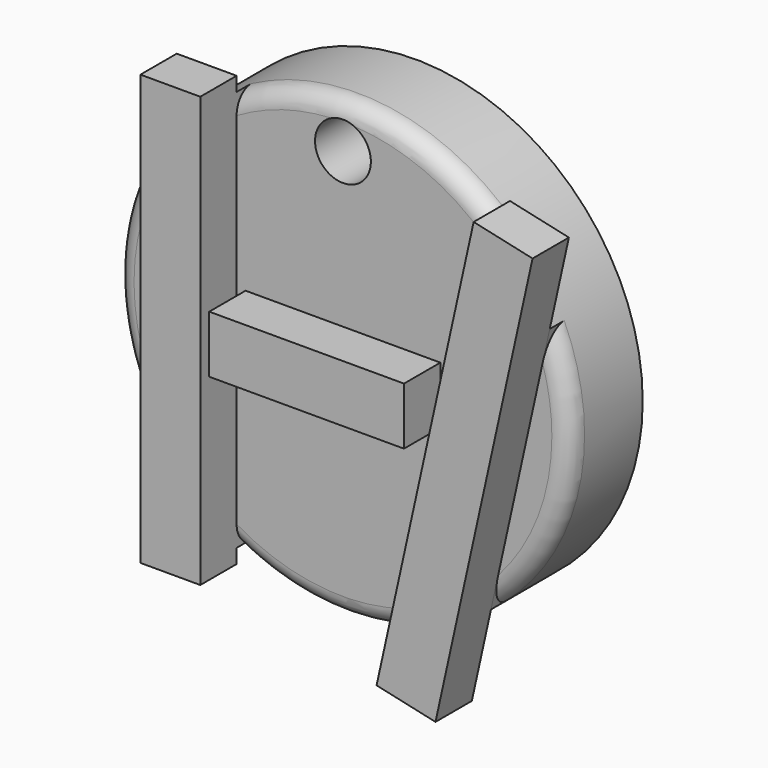
from build123d import *

# Parameters (mm, degrees)
F0_R          = 6.35
F1_DEPTH      = 2.54
F2_W          = 1.6741803847
F2_H          = 6.0100271367
F3_DEPTH      = 1.27
F4_W          = 5.4453448392
F4_H          = 0.8010258316
F5_DEPTH      = 1.27
F7_DEPTH      = 1.27
F8_R          = 0.7810995879
F9_DEPTH      = 25.4
F10_T4_ANGLE  = 60.776700367
F10_T9_ANGLE  = 70.6868696842
F10_T15_ANGLE = 108.8474457798
F10_T20_ANGLE = 95.5948420913
F10_T26_ANGLE = 35.8710937336


# Not quite as in the source:
# - a fillet or chamfer that OpenCascade refuses, or shapes differently, is made with other operations: its cross-section is extruded or revolved along the edge and cut away or added
# - a feature of the source that left no trace in its solid (it failed there, or was rolled back) is left out


with BuildPart() as f1:
    # F0 (on Front) → F1 (new body)
    with BuildSketch(Plane.XZ):
        Circle(F0_R)
    extrude(amount=F1_DEPTH)

    # F2 (on face) → F3 (join)
    with BuildSketch(Plane.XZ.offset(2.54)):
        with Locations((-3.81, 3.0050135683)):
            Rectangle(F2_W, F2_H)
        with Locations((-3.81, -3.0050135683)):
            Rectangle(F2_W, F2_H)
    extrude(amount=F3_DEPTH)

    # F4 (on face) → F5 (join)
    with BuildSketch(Plane.XZ.offset(2.54)):
        with Locations((0, 0.4005129158)):
            Rectangle(F4_W, F4_H)
        with Locations((0, -0.4005129158)):
            Rectangle(F4_W, F4_H)
    extrude(amount=F5_DEPTH)

    # F6 (on face) → F7 (join)
    with BuildSketch(Plane.XZ.offset(2.54)):
        Polygon((4.6705882996, 5.4137986153), (2.1562074386, -5.9727103966), (1.9563709538, -6.8768215956), (3.6039068937, -7.2406322096), (6.3179433579, 5.0500279438), align=None)
    extrude(amount=F7_DEPTH)

    # F8 (on face) → F9 (cut)
    with BuildSketch(Plane.XZ.offset(2.54)):
        with Locations((0, 5.1177083515)):
            Circle(F8_R)
    extrude(amount=-F9_DEPTH, mode=Mode.SUBTRACT)

    # F10: fillet of radius 0.508 on 5 edges, made by hand


with BuildPart() as f10_tool2:
    # F10_s3 → F10_t4 (revolve)
    with BuildSketch(Plane(origin=(0, 0, 0), x_dir=(0, 1, 0), z_dir=(-0.8727236144, 0, -0.4882145972))):
        with BuildLine():
            ThreePointArc((-2.032, 6.35), (-2.3912102448, 6.2012102448), (-2.54, 5.842))
            Line((-2.54, 5.842), (-2.54, 6.35))
            Line((-2.54, 6.35), (-2.032, 6.35))
        make_face()
    revolve(axis=Axis((0, -2.54, 0), (0, -1, 0)), revolution_arc=F10_T4_ANGLE)

    split(bisect_by=Plane(origin=(4.9608883724, 0, -1.0954685729), x_dir=(0, 1, 0), z_dir=(0.9764759285, 0, -0.2156264386)), keep=Keep.TOP)


with BuildPart() as f1_1:
    add(f1.part)

    # F10_t1: cut F10_tool2
    add(f10_tool2.part, mode=Mode.SUBTRACT)


with BuildPart() as f10_tool7:
    # F10_s8 → F10_t9 (revolve)
    with BuildSketch(Plane(origin=(0, 0, 0), x_dir=(0, 1, 0), z_dir=(-0.7729956778, 0, 0.6344112878))):
        with BuildLine():
            ThreePointArc((-2.032, 6.35), (-2.3912102448, 6.2012102448), (-2.54, 5.842))
            Line((-2.54, 5.842), (-2.54, 6.35))
            Line((-2.54, 6.35), (-2.032, 6.35))
        make_face()
    revolve(axis=Axis((0, -2.54, 0), (0, -1, 0)), revolution_arc=F10_T9_ANGLE)

    split(bisect_by=Plane.YZ.offset(-2.9729098076), keep=Keep.TOP)

    split(bisect_by=Plane(origin=(3.313533314, 0, -0.7316979013), x_dir=(0, 1, 0), z_dir=(-0.9764759285, 0, 0.2156264386)), keep=Keep.TOP)


with BuildPart() as f1_2:
    add(f1_1.part)

    # F10_t6: cut F10_tool7
    add(f10_tool7.part, mode=Mode.SUBTRACT)


with BuildPart() as f10_tool13:
    # F10_s14 → F10_t15 (revolve)
    with BuildSketch(Plane(origin=(0, 0, 0), x_dir=(0, 1, 0), z_dir=(0.813341715, 0, 0.581786262))):
        with BuildLine():
            ThreePointArc((-2.032, 6.35), (-2.3912102448, 6.2012102448), (-2.54, 5.842))
            Line((-2.54, 5.842), (-2.54, 6.35))
            Line((-2.54, 6.35), (-2.032, 6.35))
        make_face()
    revolve(axis=Axis((0, -2.54, 0), (0, -1, 0)), revolution_arc=F10_T15_ANGLE)

    split(bisect_by=Plane.YZ.offset(-4.6470901924), keep=Keep.BOTTOM)


with BuildPart() as f1_3:
    add(f1_2.part)

    # F10_t12: cut F10_tool13
    add(f10_tool13.part, mode=Mode.SUBTRACT)


with BuildPart() as f10_tool18:
    # F10_s19 → F10_t20 (revolve)
    with BuildSketch(Plane(origin=(0, 0, 0), x_dir=(0, 1, 0), z_dir=(0.5560518892, 0, -0.8311475781))):
        with BuildLine():
            ThreePointArc((-2.032, 6.35), (-2.3912102448, 6.2012102448), (-2.54, 5.842))
            Line((-2.54, 5.842), (-2.54, 6.35))
            Line((-2.54, 6.35), (-2.032, 6.35))
        make_face()
    revolve(axis=Axis((0, -2.54, 0), (0, -1, 0)), revolution_arc=F10_T20_ANGLE)

    split(bisect_by=Plane.YZ.offset(-2.9729098076), keep=Keep.TOP)

    split(bisect_by=Plane(origin=(3.313533314, 0, -0.7316979013), x_dir=(0, 1, 0), z_dir=(-0.9764759285, 0, 0.2156264386)), keep=Keep.TOP)


with BuildPart() as f1_4:
    add(f1_3.part)

    # F10_t17: cut F10_tool18
    add(f10_tool18.part, mode=Mode.SUBTRACT)


with BuildPart() as f10_tool24:
    # F10_s25 → F10_t26 (revolve)
    with BuildSketch(Plane.XY):
        with BuildLine():
            ThreePointArc((6.35, -2.032), (6.2012102448, -2.3912102448), (5.842, -2.54))
            Line((5.842, -2.54), (6.35, -2.54))
            Line((6.35, -2.54), (6.35, -2.032))
        make_face()
    revolve(axis=Axis((0, -2.54, 0), (0, -1, 0)), revolution_arc=F10_T26_ANGLE)

    split(bisect_by=Plane(origin=(4.9608883724, 0, -1.0954685729), x_dir=(0, 1, 0), z_dir=(0.9764759285, 0, -0.2156264386)), keep=Keep.TOP)


with BuildPart() as f1_5:
    add(f1_4.part)

    # F10_t23: cut F10_tool24
    add(f10_tool24.part, mode=Mode.SUBTRACT)


solid = f1_5.part
